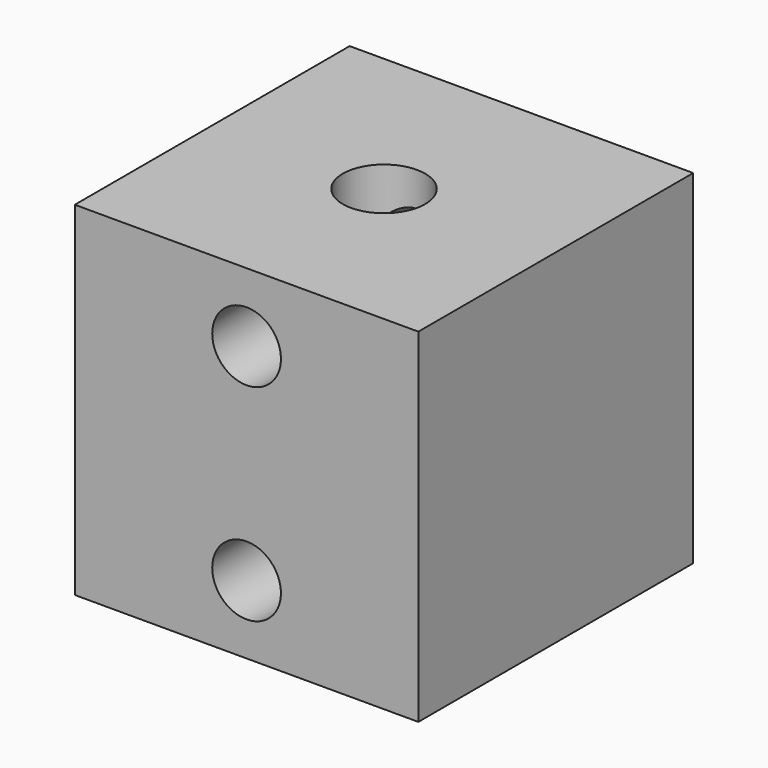
from build123d import *

# Parameters (mm, degrees)
F0_W     = 25
F0_H     = 25
F1_DEPTH = 25
F3_D     = 6
F5_D     = 5
F7_D     = 5


with BuildPart() as f1:
    # F0 (on Top) → F1 (new body)
    with BuildSketch(Plane.XY):
        with Locations((-12.5, 12.5)):
            Rectangle(F0_W, F0_H)
    extrude(amount=F1_DEPTH)

    # F3 (through all)
    with Locations(Plane.XY.offset(25)):
        with Locations((-12.5, 12.5)):
            Hole(F3_D / 2)

    # F5 (through all)
    with Locations(Plane.XZ):
        with Locations((-12.5, 20)):
            Hole(F5_D / 2)

    # F7 (through all)
    with Locations(Plane.XZ):
        with Locations((-12.5, 5)):
            Hole(F7_D / 2)


solid = f1.part
